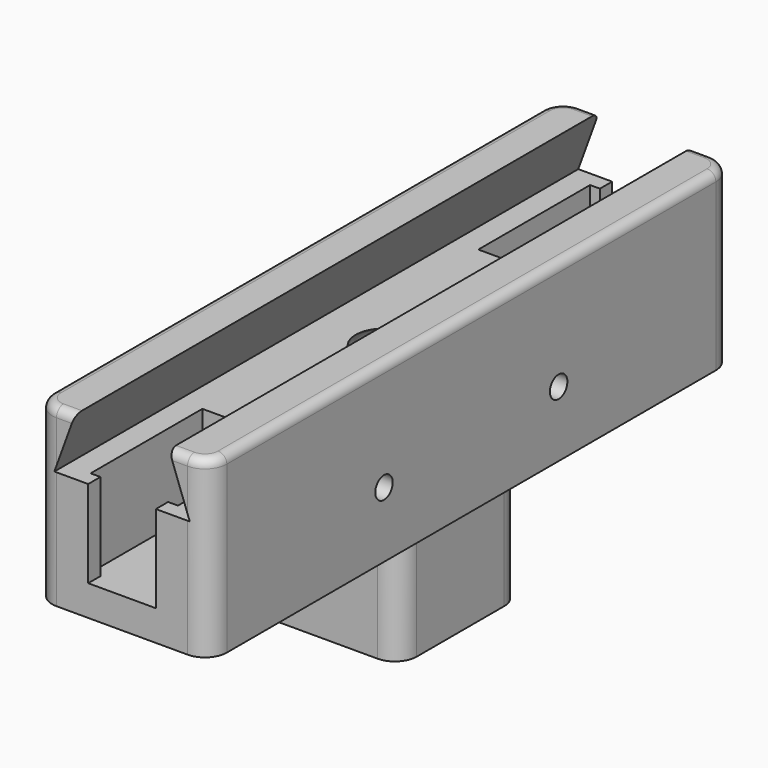
from build123d import *

# Parameters (mm, degrees)
F0_W           = 40
F0_H           = 27
F1_DEPTH       = 150
F2_W           = 15.5
F2_H           = 3.5
F3_DEPTH       = 20
F5_W           = 35
F5_H           = 35
F5_R           = 8.5
F6_DEPTH       = 25
F4_R           = 8.5
F7_DEPTH       = 25
F8_R           = 5.5
F9_DEPTH       = 52.001
F10_S5_R       = 8.5
F10_T6_DEPTH   = 14
F11_R          = 5
F13_DEPTH      = 150
F14_T1_DEPTH   = 65
F14_T3_DEPTH   = 37.5
F15_R          = 2
F16_R          = 2.5
F17_DEPTH      = 20.001
F17_DEPTH_BACK = 25
F18_SIZE       = 3


# Not quite as in the source:
# - a fillet or chamfer that OpenCascade refuses, or shapes differently, is made with other operations: its cross-section is extruded or revolved along the edge and cut away or added


with BuildPart() as f1:
    # F0 (on Front) → F1 (new body)
    with BuildSketch(Plane.XZ):
        Rectangle(F0_W, F0_H)
    extrude(amount=F1_DEPTH)

    # F2 (on face) → F3 (cut)
    with BuildSketch(Plane.XY.offset(13.5)):
        with Locations((0, -1.75)):
            Rectangle(F2_W, F2_H)
        Polygon((-7.75, -3.5), (-10, -3.5), (-10, -35.5), (10, -35.5), (10, -3.5), (7.75, -3.5), align=None)
        Polygon((-10, -146.5), (-7.75, -146.5), (7.75, -146.5), (10, -146.5), (10, -114.5), (-10, -114.5), align=None)
        with Locations((0, -148.25)):
            Rectangle(F2_W, F2_H)
    extrude(amount=-F3_DEPTH, mode=Mode.SUBTRACT)

    # F5 (on face) → F6 (join)
    with BuildSketch(Plane(origin=(0, 0, -13.5), x_dir=(1, 0, 0), z_dir=(0, 0, -1))):
        with Locations((0, 75)):
            Rectangle(F5_W, F5_H)
        with Locations((0, 75)):
            Circle(F5_R, mode=Mode.SUBTRACT)
    extrude(amount=F6_DEPTH)

    # F4 (on face) → F7 (cut)
    with BuildSketch(Plane(origin=(0, 0, -13.5), x_dir=(1, 0, 0), z_dir=(0, 0, -1))):
        with Locations((0, 75)):
            Circle(F4_R)
    extrude(amount=-F7_DEPTH, mode=Mode.SUBTRACT)

    # F8 (on face) → F9 (cut, through all)
    with BuildSketch(Plane.XY.offset(13.5)):
        with Locations((0, -75)):
            Circle(F8_R)
    extrude(amount=-F9_DEPTH, mode=Mode.SUBTRACT)

    # F10: chamfer of 3 on 1 edges, made by hand


with BuildPart() as f10_tool2:
    # F10_s3 → F10_t4 (revolve)
    with BuildSketch(Plane.XZ.offset(75)):
        Polygon((5.5, 14.5), (8.5, 11.5), (5.5, 11.5), align=None)
    revolve(axis=Axis((0, -75, 11.5), (0, 0, 1)))

    # F10_s5 → F10_t6 (intersect, symmetric)
    with BuildSketch(Plane.XY.offset(13)):
        with Locations((0, -75)):
            Circle(F10_S5_R)
    extrude(amount=F10_T6_DEPTH, both=True, mode=Mode.INTERSECT)


with BuildPart() as f1_1:
    add(f1.part)

    # F10_t1: cut F10_tool2
    add(f10_tool2.part, mode=Mode.SUBTRACT)

    # F11
    f11_edges = [f1_1.edges().sort_by_distance(p)[0] for p in [
        (-8.5, -75, 11.5),
    ]]
    fillet(f11_edges, radius=F11_R)

    # F12 (on Front) → F13 (join, through all)
    with BuildSketch(Plane.XZ):
        Polygon((10.7683869545, 26.5), (15.5, 13.5), (20, 13.5), (20, 26.5), align=None)
        Polygon((-20, 26.5), (-20, 13.5), (-15.5, 13.5), (-10.7683869545, 26.5), align=None)
    extrude(amount=F13_DEPTH)

    # F14: fillet of radius 5 on 8 edges, made by hand

    # F14_s2 → F14_t1 (cut)
    with BuildSketch(Plane.XY.offset(-26)):
        with BuildLine():
            ThreePointArc((-20, -145), (-18.5355339059, -148.5355339059), (-15, -150))
            Line((-15, -150), (-20, -150))
            Line((-20, -150), (-20, -145))
        make_face()
        with BuildLine():
            ThreePointArc((20, -145), (18.5355339059, -148.5355339059), (15, -150))
            Line((15, -150), (20, -150))
            Line((20, -150), (20, -145))
        make_face()
        with BuildLine():
            ThreePointArc((20, -5), (18.5355339059, -1.4644660941), (15, 0))
            Line((15, 0), (20, 0))
            Line((20, 0), (20, -5))
        make_face()
        with BuildLine():
            ThreePointArc((-20, -5), (-18.5355339059, -1.4644660941), (-15, 0))
            Line((-15, 0), (-20, 0))
            Line((-20, 0), (-20, -5))
        make_face()
    extrude(amount=F14_T1_DEPTH, mode=Mode.SUBTRACT)

    # F14_s4 → F14_t3 (cut)
    with BuildSketch(Plane.XY.offset(-51)):
        with BuildLine():
            ThreePointArc((12.5, -57.5), (16.0355339059, -58.9644660941), (17.5, -62.5))
            Line((17.5, -62.5), (17.5, -57.5))
            Line((17.5, -57.5), (12.5, -57.5))
        make_face()
        with BuildLine():
            ThreePointArc((12.5, -92.5), (16.0355339059, -91.0355339059), (17.5, -87.5))
            Line((17.5, -87.5), (17.5, -92.5))
            Line((17.5, -92.5), (12.5, -92.5))
        make_face()
        with BuildLine():
            ThreePointArc((-17.5, -62.5), (-16.0355339059, -58.9644660941), (-12.5, -57.5))
            Line((-12.5, -57.5), (-17.5, -57.5))
            Line((-17.5, -57.5), (-17.5, -62.5))
        make_face()
        with BuildLine():
            ThreePointArc((-12.5, -92.5), (-16.0355339059, -91.0355339059), (-17.5, -87.5))
            Line((-17.5, -87.5), (-17.5, -92.5))
            Line((-17.5, -92.5), (-12.5, -92.5))
        make_face()
    extrude(amount=F14_T3_DEPTH, mode=Mode.SUBTRACT)

    # F15
    f15_edges = [f1_1.edges().sort_by_distance(p)[0] for p in [
        (-12.884193, -150, 26.5),
        (12.884193, -150, 26.5),
    ]]
    fillet(f15_edges, radius=F15_R)

    # F16 (on Right) → F17 (cut, two sides)
    with BuildSketch(Plane.YZ) as f17_sk:
        with Locations((-100, 1.5)):
            Circle(F16_R)
        with Locations((-50, 1.5)):
            Circle(F16_R)
    extrude(amount=-F17_DEPTH, mode=Mode.SUBTRACT)
    extrude(f17_sk.sketch, amount=F17_DEPTH_BACK, mode=Mode.SUBTRACT)

    # F18
    f18_edges = [f1_1.edges().sort_by_distance(p)[0] for p in [
        (-20, -52.5, 1.5),
        (-20, -102.5, 1.5),
    ]]
    chamfer(f18_edges, length=F18_SIZE)


solid = f1_1.part
